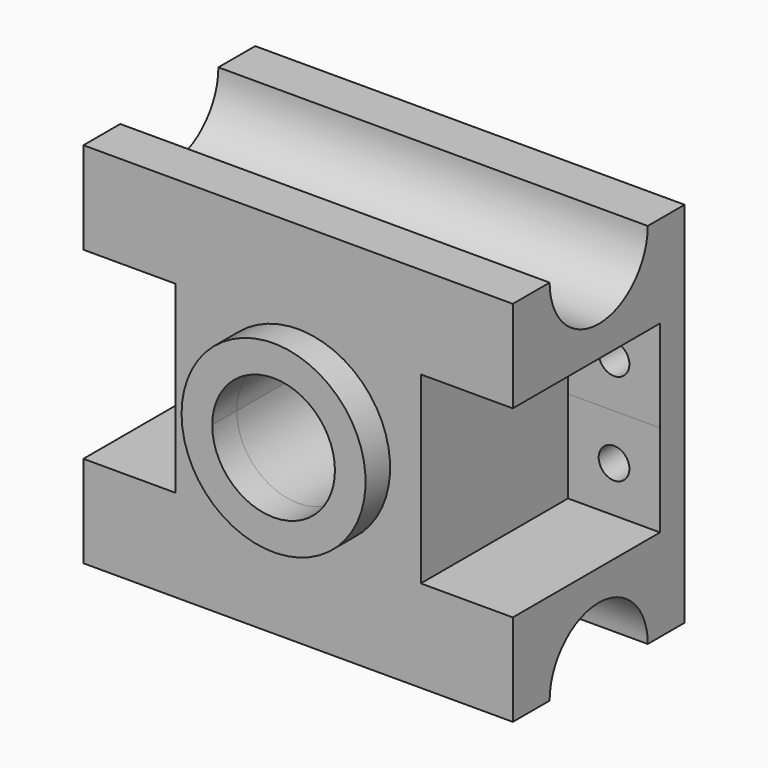
from build123d import *

# Parameters (mm, degrees)
F0_W      = 140
F0_H      = 60
F1_DEPTH  = 35
F3_DEPTH  = 140.001
F4_W      = 30
F4_H      = 30
F5_DEPTH  = 60
F6_R      = 20
F7_DEPTH  = 72.1
F9_DEPTH  = 10
F11_DEPTH = 25
F12_R     = 5
F13_DEPTH = 25


# Not quite as in the source:
# - a pattern or mirror of a feature is missing from the dataset's text; its kind, count and spacing are read off the source's solid


with BuildPart() as f1:
    # F0 (on Front) → F1 (new body, symmetric)
    with BuildSketch(Plane.XZ):
        Rectangle(F0_W, F0_H)
    extrude(amount=F1_DEPTH, both=True)

    # F2 (on face) → F3 (cut, through all)
    with BuildSketch(Plane.YZ.offset(70)):
        with BuildLine():
            Line((-20, -30), (20, -30))
            ThreePointArc((20, -30), (0, -10), (-20, -30))
        make_face()
        with BuildLine():
            ThreePointArc((-20, -30), (0, -50), (20, -30))
            Line((20, -30), (-20, -30))
        make_face()
    extrude(amount=-F3_DEPTH, mode=Mode.SUBTRACT)

    # F4 (on face) → F5 (cut)
    with BuildSketch(Plane.XZ.offset(35)):
        with Locations((55, 15)):
            Rectangle(F4_W, F4_H)
    f5 = extrude(amount=-F5_DEPTH, mode=Mode.SUBTRACT)

    # F5_copies: F5 across plane
    add(f5.mirror(Plane(origin=(0, 0, 0), x_dir=(0, 0, -1), z_dir=(-1, 0, 0))), mode=Mode.SUBTRACT)

    # F6 (on face) → F7 (cut)
    with BuildSketch(Plane.XZ.offset(35)):
        with Locations((0, 30)):
            Circle(F6_R)
    extrude(amount=-F7_DEPTH, mode=Mode.SUBTRACT)

    # F8 (on face) → F9 (join)
    with BuildSketch(Plane.XZ.offset(35)):
        with BuildLine():
            Line((0, 30), (-30, 30))
            ThreePointArc((-30, 30), (0, 0), (30, 30))
            Line((30, 30), (0, 30))
        make_face()
    extrude(amount=F9_DEPTH)

    # F10 (on face) → F11 (cut)
    with BuildSketch(Plane(origin=(0, -35, 0), x_dir=(-1, 0, 0), z_dir=(0, 1, 0))):
        with BuildLine():
            ThreePointArc((-20, 30), (0, 10), (20, 30))
            Line((20, 30), (-20, 30))
        make_face()
    extrude(amount=-F11_DEPTH, mode=Mode.SUBTRACT)

    # F12 (on face) → F13 (cut)
    with BuildSketch(Plane.XZ.offset(-25)):
        with Locations((55, 15)):
            Circle(F12_R)
    f13 = extrude(amount=-F13_DEPTH, mode=Mode.SUBTRACT)

    # F13_copies: F13 across plane
    add(f13.mirror(Plane(origin=(0, 0, 0), x_dir=(0, 0, -1), z_dir=(-1, 0, 0))), mode=Mode.SUBTRACT)

    # F15: F1 across plane


with BuildPart() as f1_1:
    add(f1.part)
    add(f1.part.mirror(Plane.XY.offset(30)))


solid = f1_1.part
